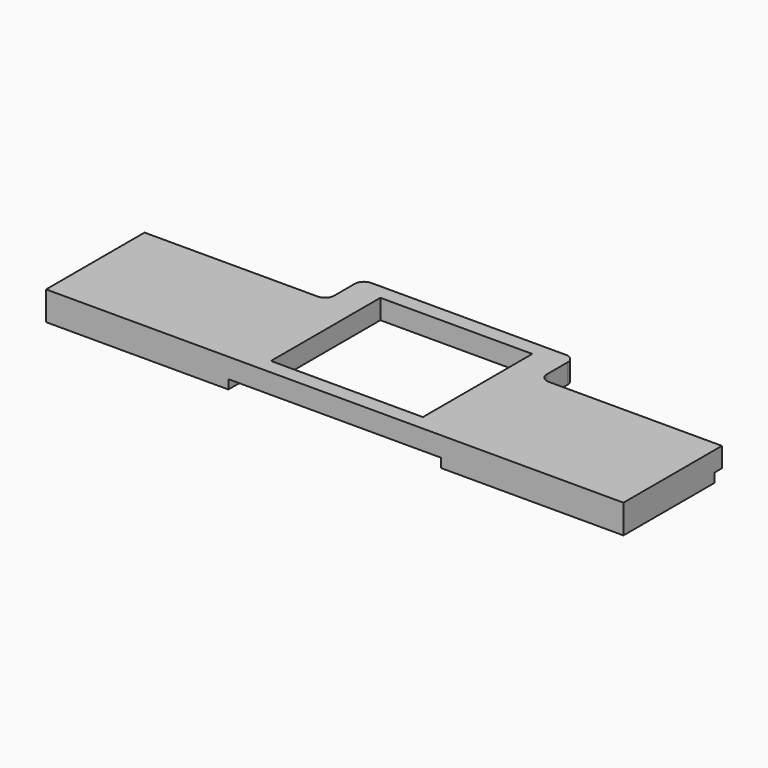
from build123d import *

# Parameters (mm, degrees)
F0_W     = 120
F0_H     = 6
F0_W_2   = 6
F0_H_2   = 23
F0_H_3   = 75
F1_DEPTH = 19
F2_DEPTH = 6
F3_R     = 6
F4_R     = 2.5
F5_DEPTH = 25


with BuildPart() as f1:
    # F0 (on Top) → F1 (new body)
    with BuildSketch(Plane.XY):
        with Locations((29.2149764299, 55.6197040975)):
            Rectangle(F0_W, F0_H)
        with Locations((92.2149764299, 70.1197040975)):
            Rectangle(F0_W_2, F0_H_2)
        with Locations((92.2149764299, 55.6197040975)):
            Rectangle(F0_W_2, F0_H)
        with Locations((29.2149764299, 15.1197040975)):
            Rectangle(F0_W, F0_H_3)
        Polygon((109.2149764299, 58.6197040975), (95.2149764299, 58.6197040975), (95.2149764299, 52.6197040975), (89.2149764299, 52.6197040975), (89.2149764299, -22.3802959025), (159.2149764299, -22.3802959025), (159.2149764299, -12.3802959025), (109.2149764299, -12.3802959025), align=None)
        Polygon((89.2149764299, 87.6197040975), (89.2149764299, 81.6197040975), (95.2149764299, 81.6197040975), (159.2149764299, 81.6197040975), (159.2149764299, 87.6197040975), align=None)
        Polygon((159.2149764299, 87.6197040975), (159.2149764299, 81.6197040975), (223.2149764299, 81.6197040975), (229.2149764299, 81.6197040975), (229.2149764299, 87.6197040975), align=None)
        Polygon((159.2149764299, -12.3802959025), (159.2149764299, -22.3802959025), (229.2149764299, -22.3802959025), (229.2149764299, 52.6197040975), (229.2137485743, 52.6197040975), (223.2149764299, 52.6197040975), (223.2149764299, 58.6197040975), (209.2149764299, 58.6197040975), (209.2149764299, -12.3802959025), align=None)
        with Locations((226.2149764299, 70.1197040975)):
            Rectangle(F0_W_2, F0_H_2)
        with Locations((289.2149764299, 15.1197040975)):
            Rectangle(F0_W, F0_H_3)
        Polygon((229.2149764299, 58.6197040975), (223.2149764299, 58.6197040975), (223.2149764299, 52.6197040975), (229.2137485743, 52.6197040975), (229.2149764299, 52.6197040975), align=None)
        with Locations((289.2149764299, 55.6197040975)):
            Rectangle(F0_W, F0_H)
        Polygon((95.2149764299, 81.6197040975), (95.2149764299, 58.6197040975), (109.2149764299, 58.6197040975), (109.2149764299, 77.6197040975), (159.2149764299, 77.6197040975), (159.2149764299, 81.6197040975), align=None)
        Polygon((223.2149764299, 81.6197040975), (159.2149764299, 81.6197040975), (159.2149764299, 77.6197040975), (209.2149764299, 77.6197040975), (209.2149764299, 58.6197040975), (223.2149764299, 58.6197040975), align=None)
    extrude(amount=F1_DEPTH)

    # F0 (on Top) → F2 (cut)
    with BuildSketch(Plane.XY):
        with Locations((29.2149764299, 55.6197040975)):
            Rectangle(F0_W, F0_H)
        with Locations((92.2149764299, 55.6197040975)):
            Rectangle(F0_W_2, F0_H)
        with Locations((289.2149764299, 55.6197040975)):
            Rectangle(F0_W, F0_H)
        with Locations((92.2149764299, 70.1197040975)):
            Rectangle(F0_W_2, F0_H_2)
        Polygon((89.2149764299, 87.6197040975), (89.2149764299, 81.6197040975), (95.2149764299, 81.6197040975), (159.2149764299, 81.6197040975), (159.2149764299, 87.6197040975), align=None)
        Polygon((159.2149764299, 87.6197040975), (159.2149764299, 81.6197040975), (223.2149764299, 81.6197040975), (229.2149764299, 81.6197040975), (229.2149764299, 87.6197040975), align=None)
        with Locations((226.2149764299, 70.1197040975)):
            Rectangle(F0_W_2, F0_H_2)
        Polygon((229.2149764299, 58.6197040975), (223.2149764299, 58.6197040975), (223.2149764299, 52.6197040975), (229.2137485743, 52.6197040975), (229.2149764299, 52.6197040975), align=None)
        Polygon((159.2149764299, -12.3802959025), (159.2149764299, -22.3802959025), (229.2149764299, -22.3802959025), (229.2149764299, 52.6197040975), (229.2137485743, 52.6197040975), (223.2149764299, 52.6197040975), (223.2149764299, 58.6197040975), (209.2149764299, 58.6197040975), (209.2149764299, -12.3802959025), align=None)
        Polygon((109.2149764299, 58.6197040975), (95.2149764299, 58.6197040975), (95.2149764299, 52.6197040975), (89.2149764299, 52.6197040975), (89.2149764299, -22.3802959025), (159.2149764299, -22.3802959025), (159.2149764299, -12.3802959025), (109.2149764299, -12.3802959025), align=None)
        Polygon((223.2149764299, 81.6197040975), (159.2149764299, 81.6197040975), (159.2149764299, 77.6197040975), (209.2149764299, 77.6197040975), (209.2149764299, 58.6197040975), (223.2149764299, 58.6197040975), align=None)
        Polygon((95.2149764299, 81.6197040975), (95.2149764299, 58.6197040975), (109.2149764299, 58.6197040975), (109.2149764299, 77.6197040975), (159.2149764299, 77.6197040975), (159.2149764299, 81.6197040975), align=None)
    extrude(amount=F2_DEPTH, mode=Mode.SUBTRACT)

    # F3
    f3_edges = [f1.edges().sort_by_distance(p)[0] for p in [
        (229.214976, 58.619704, 12.5),
        (229.214976, 87.619704, 12.5),
        (89.214976, 87.619704, 12.5),
        (89.214976, 58.619704, 12.5),
    ]]
    fillet(f3_edges, radius=F3_R)

    # F4 (on face) → F5 (cut)
    with BuildSketch(Plane(origin=(-30.7850235701, 0, 0), x_dir=(0, -1, 0), z_dir=(-1, 0, 0))):
        with Locations((-32.6197040975, 9.5)):
            Circle(F4_R)
        with Locations((2.3802959025, 9.5)):
            Circle(F4_R)
    extrude(amount=-F5_DEPTH, mode=Mode.SUBTRACT)


solid = f1.part
